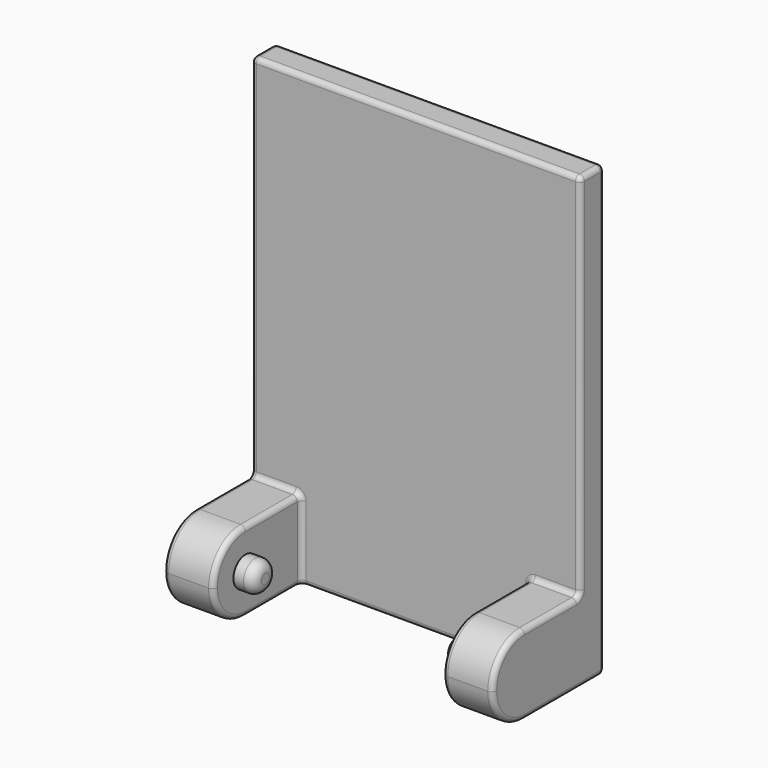
from build123d import *

# Parameters (mm, degrees)
F0_W     = 33
F0_H     = 45
F1_DEPTH = 3
F2_W     = 5
F2_H     = 8
F3_DEPTH = 11
F4_R     = 1.5
F5_DEPTH = 2
F6_R     = 1
F7_R     = 1.5
F8_DEPTH = 2
F9_R     = 1
F10_R    = 3.99999
F11_R    = 0.5


# Not quite as in the source:
# - a fillet or chamfer is up to 0.001 mm smaller than in the source, because OpenCascade refuses the exact size


with BuildPart() as f1:
    # F0 (on Front) → F1 (new body)
    with BuildSketch(Plane.XZ):
        with Locations((16.5, 22.5)):
            Rectangle(F0_W, F0_H)
    extrude(amount=-F1_DEPTH)

    # F2 (on face) → F3 (join)
    with BuildSketch(Plane.XZ):
        with Locations((2.5, 4)):
            Rectangle(F2_W, F2_H)
        with Locations((30.5, 4)):
            Rectangle(F2_W, F2_H)
    extrude(amount=F3_DEPTH)

    # F4 (on face) → F5 (join)
    with BuildSketch(Plane.YZ.offset(5)):
        with Locations((-7, 4)):
            Circle(F4_R)
    extrude(amount=F5_DEPTH)

    # F6
    f6_edges = [f1.edges().sort_by_distance(p)[0] for p in [
        (7, -8.5, 4),
    ]]
    fillet(f6_edges, radius=F6_R)

    # F7 (on face) → F8 (join)
    with BuildSketch(Plane(origin=(28, 0, 0), x_dir=(0, -1, 0), z_dir=(-1, 0, 0))):
        with Locations((7, 4)):
            Circle(F7_R)
    extrude(amount=F8_DEPTH)

    # F9
    f9_edges = [f1.edges().sort_by_distance(p)[0] for p in [
        (26, -5.5, 4),
    ]]
    fillet(f9_edges, radius=F9_R)

    # F10 (radius 4 in the source; OpenCascade refuses exactly that, so slightly less here)
    f10_edges = [f1.edges().sort_by_distance(p)[0] for p in [
        (2.5, -11, 8),
        (2.5, -11, 0),
        (30.5, -11, 8),
        (30.5, -11, 0),
    ]]
    fillet(f10_edges, radius=F10_R)

    # F11
    f11_edges = [f1.edges().sort_by_distance(p)[0] for p in [
        (0, 0, 26.5),
        (16.5, 0, 45),
        (33, 0, 26.5),
        (33, 1.5, 45),
        (33, 3, 22.5),
        (0, 1.5, 45),
        (16.5, 3, 45),
        (0, 3, 22.5),
        (16.5, 0, 0),
        (28, 0, 4),
        (0, -2.000005, 0),
        (0, -9.82843, 1.17157),
        (0, -3.500005, 8),
        (5, -9.82843, 1.17157),
        (5, -3.500005, 0),
        (16.5, 3, 0),
        (5, -3.500005, 8),
        (2.5, 0, 8),
        (28, -3.500005, 8),
        (28, -9.82843, 6.82843),
        (28, -11, 4),
        (28, -3.500005, 0),
        (28, -9.82843, 1.17157),
        (33, -3.500005, 8),
        (30.5, 0, 8),
        (33, -9.82843, 6.82843),
        (5, 0, 4),
        (33, -11, 4),
        (33, -2.000005, 0),
        (33, -9.82843, 1.17157),
        (5, -11, 4),
        (5, -9.82843, 6.82843),
        (0, -11, 4),
        (0, -9.82843, 6.82843),
    ]]
    fillet(f11_edges, radius=F11_R)


solid = f1.part
